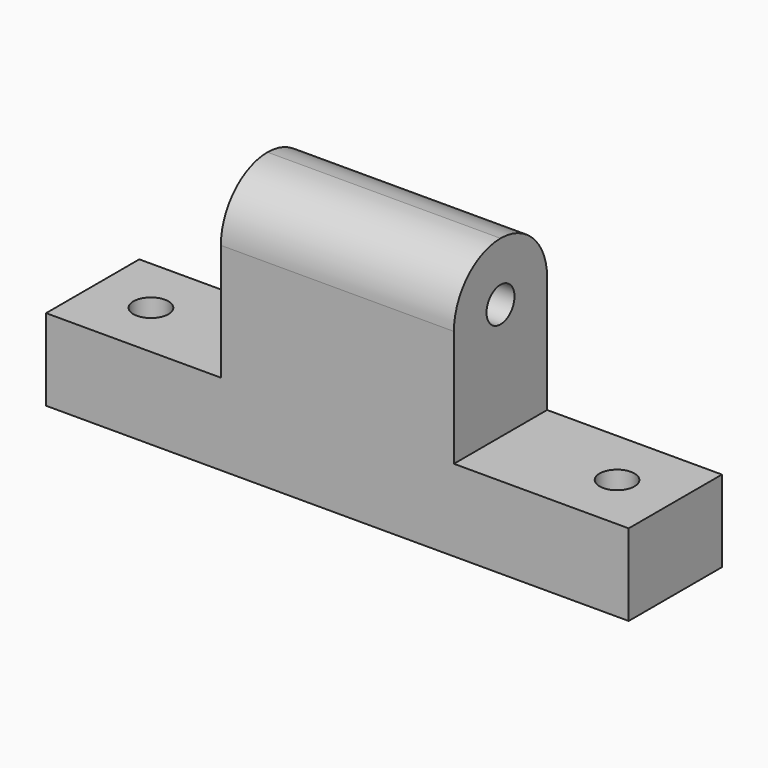
from build123d import *

# Parameters (mm, degrees)
F0_W      = 50
F0_H      = 10
F1_DEPTH  = 7
F2_W      = 20
F2_H      = 10
F4_DEPTH  = 15
F5_R      = 4.99999
F3_R      = 1.5
F6_DEPTH  = 25
F7_R      = 1.5
F8_DEPTH  = 50
F10_W     = 10
F10_H     = 10
F11_DEPTH = 25


# Not quite as in the source:
# - a fillet or chamfer is up to 0.001 mm smaller than in the source, because OpenCascade refuses the exact size


with BuildPart() as f1:
    # F0 (on Top) → F1 (new body)
    with BuildSketch(Plane.XY):
        with Locations((25, 5)):
            Rectangle(F0_W, F0_H)
    extrude(amount=F1_DEPTH)

    # F2 (on face) → F4 (join)
    with BuildSketch(Plane.XY.offset(7)):
        with Locations((25, 5)):
            Rectangle(F2_W, F2_H)
    extrude(amount=F4_DEPTH)

    # F5 (radius 5 in the source; OpenCascade refuses exactly that, so slightly less here)
    f5_edges = [f1.edges().sort_by_distance(p)[0] for p in [
        (25, 10, 22),
        (25, 0, 22),
    ]]
    fillet(f5_edges, radius=F5_R)

    # F3 (on face) → F6 (cut)
    with BuildSketch(Plane.XY.offset(7)):
        with Locations((45, 5)):
            Circle(F3_R)
        with Locations((5, 5)):
            Circle(F3_R)
    extrude(amount=-F6_DEPTH, mode=Mode.SUBTRACT)

    # F7 (on face) → F8 (cut)
    with BuildSketch(Plane.YZ.offset(35)):
        with Locations((5, 17)):
            Circle(F7_R)
    extrude(amount=-F8_DEPTH, mode=Mode.SUBTRACT)


with BuildPart() as f9_1:
    # F9: copy of F1
    add(f1.part.moved(Location((0, 0, 40))))

    # F10 (on face) → F11 (cut)
    with BuildSketch(Plane.XY.offset(47)):
        with Locations((25, 5)):
            Rectangle(F10_W, F10_H)
    extrude(amount=F11_DEPTH, mode=Mode.SUBTRACT)


solid = f1.part
